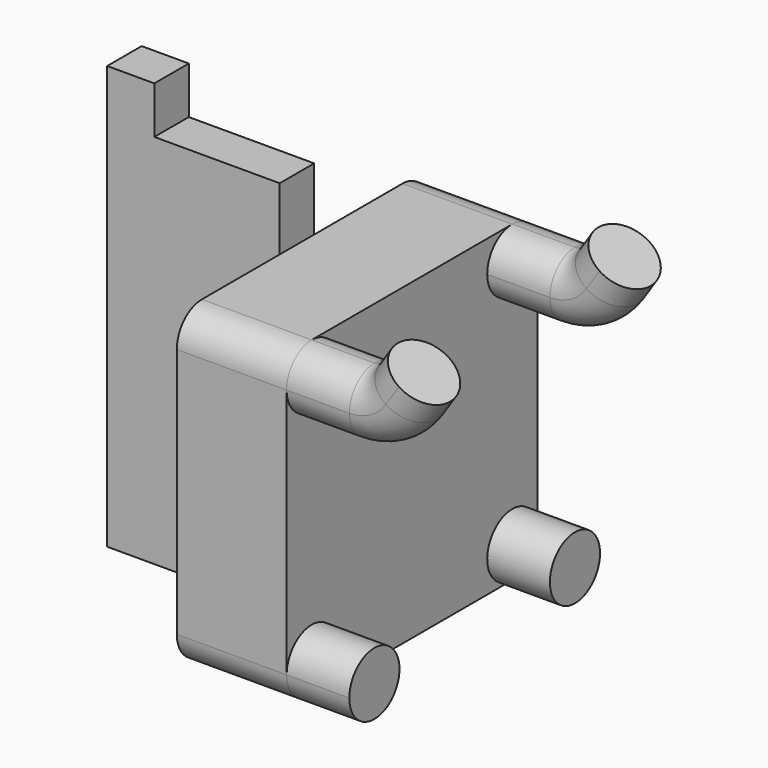
from build123d import *

# Parameters (mm, degrees)
F0_W      = 31.75
F0_H      = 31.75
F1_DEPTH  = 11.1252
F10_DEPTH = 6.35
F11_R     = 3.1749
F12_W     = 4.36372
F12_H     = 6.35
F12_H_2   = 31.75
F13_DEPTH = 17.4752
F14_W     = 4.7752
F14_H     = 4.36372
F15_DEPTH = 4.7752


# Not quite as in the source:
# - a fillet or chamfer is up to 0.001 mm smaller than in the source, because OpenCascade refuses the exact size


with BuildPart() as f1:
    # F0 (on Right) → F1 (new body)
    with BuildSketch(Plane.YZ):
        Rectangle(F0_W, F0_H)
    extrude(amount=F1_DEPTH)

    # F6: sweep along a path in F5
    with BuildLine(Plane.XZ.offset(12.7)) as f6_path:
        Line((11.1252, 9.525), (17.4752, 9.525))
        ThreePointArc((17.4752, 9.525), (21.0785384003, 10.4308096264), (23.8252, 12.9328865162))
        Line((23.8252, 12.9328865162), (25.1507334947, 14.9312034475))
    # F2 (on face) → F6 (sweep)
    with BuildSketch(Plane.YZ.offset(11.1252)):
        with BuildLine():
            ThreePointArc((-15.875, 12.7), (-12.7, 9.525), (-9.525, 12.7))
            ThreePointArc((-9.525, 12.7), (-10.4549359718, 14.9450640323), (-12.7000000057, 15.875))
            ThreePointArc((-12.7000000057, 15.875), (-14.9450640323, 14.9450640282), (-15.875, 12.7))
        make_face()
    sweep(path=f6_path.line)

    # F9: F1 across plane


with BuildPart() as f1_1:
    add(f1.part)
    add(f1.part.mirror(Plane(origin=(0, 0, 15.875), x_dir=(1, 0, 0), z_dir=(0, -1, 0))))

    # F2 (on face) → F10 (join)
    with BuildSketch(Plane.YZ.offset(11.1252)):
        with BuildLine():
            ThreePointArc((-9.525, -12.7), (-12.7, -9.525), (-15.875, -12.7))
            ThreePointArc((-15.875, -12.7), (-14.9450640303, -14.9450640303), (-12.7, -15.875))
            ThreePointArc((-12.7, -15.875), (-10.4549359697, -14.9450640303), (-9.525, -12.7))
        make_face()
        with BuildLine():
            ThreePointArc((12.7, -15.875), (14.9450640303, -14.9450640303), (15.875, -12.7))
            ThreePointArc((15.875, -12.7), (10.4549359697, -10.4549359697), (12.7, -15.875))
        make_face()
    extrude(amount=F10_DEPTH)

    # F11 (radius 3.175 in the source; OpenCascade refuses exactly that, so slightly less here)
    f11_edges = [f1_1.edges().sort_by_distance(p)[0] for p in [
        (5.5626, -15.875, 15.875),
        (5.5626, -15.875, -15.875),
        (5.5626, 15.875, -15.875),
        (5.5626, 15.875, 15.875),
    ]]
    fillet(f11_edges, radius=F11_R)

    # F12 (on face) → F13 (join)
    with BuildSketch(Plane(origin=(0, 0, 0), x_dir=(0, -1, 0), z_dir=(-1, 0, 0))):
        with Locations((0.6621663562, 19.05)):
            Rectangle(F12_W, F12_H)
        with Locations((0.6621663562, 0)):
            Rectangle(F12_W, F12_H_2)
    extrude(amount=F13_DEPTH)

    # F14 (on face) → F15 (join)
    with BuildSketch(Plane.XY.offset(22.225)):
        with Locations((-15.0876, -0.6621663562)):
            Rectangle(F14_W, F14_H)
    extrude(amount=F15_DEPTH)


solid = f1_1.part
